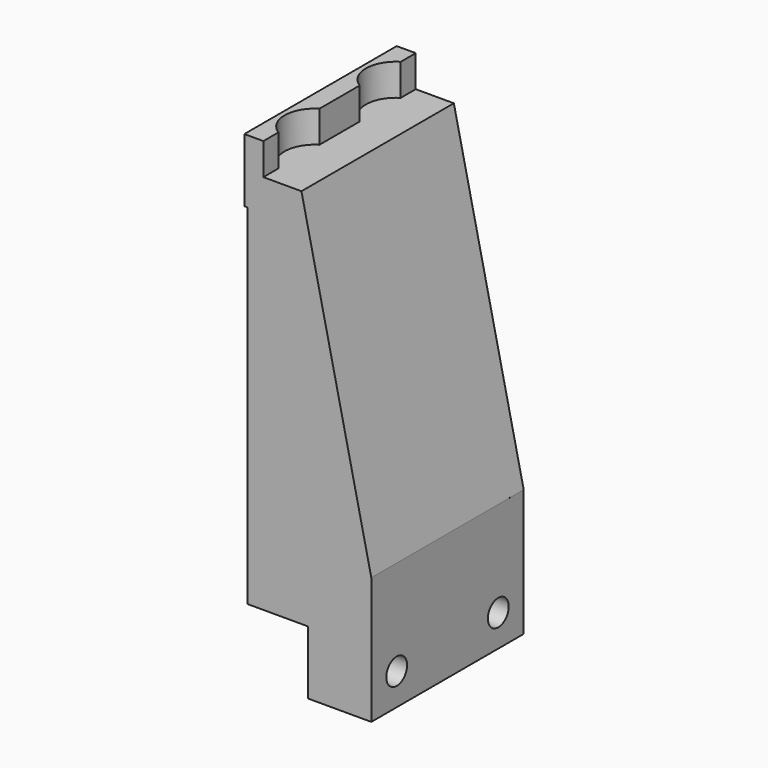
from build123d import *

# Parameters (mm, degrees)
F0_W      = 20
F0_H      = 70
F1_DEPTH  = 30
F2_W      = 30
F2_H      = 10
F3_DEPTH  = 10
F4_R      = 2.05
F5_DEPTH  = 10
F6_W      = 11
F6_H      = 30
F7_DEPTH  = 50
F9_DEPTH  = 5
F10_SIZE2 = 10.99999
F10_SIZE  = 49.99999
F11_W     = 30
F11_H     = 55
F12_DEPTH = 0.5


# Not quite as in the source:
# - a fillet or chamfer is up to 0.001 mm smaller than in the source, because OpenCascade refuses the exact size


with BuildPart() as f1:
    # F0 (on Front) → F1 (new body)
    with BuildSketch(Plane.XZ):
        with Locations((-10, 35)):
            Rectangle(F0_W, F0_H)
    extrude(amount=F1_DEPTH)

    # F2 (on face) → F3 (cut)
    with BuildSketch(Plane(origin=(-20, 0, 0), x_dir=(0, -1, 0), z_dir=(-1, 0, 0))):
        with Locations((15, 5)):
            Rectangle(F2_W, F2_H)
    extrude(amount=-F3_DEPTH, mode=Mode.SUBTRACT)

    # F4 (on face) → F5 (cut, through all)
    with BuildSketch(Plane(origin=(-10, 0, 0), x_dir=(0, -1, 0), z_dir=(-1, 0, 0))):
        with Locations((5, 5)):
            Circle(F4_R)
        with Locations((25, 5)):
            Circle(F4_R)
    extrude(amount=-F5_DEPTH, mode=Mode.SUBTRACT)

    # F6 (on face) → F7 (cut)
    with BuildSketch(Plane.XY.offset(70)):
        with Locations((-5.5, -15)):
            Rectangle(F6_W, F6_H)
    extrude(amount=-F7_DEPTH, mode=Mode.SUBTRACT)

    # F8 (on face) → F9 (join)
    with BuildSketch(Plane.XY.offset(70)):
        with BuildLine():
            ThreePointArc((-17, -11.0388736054), (-19.25, -7), (-17, -2.9611263946))
            Line((-17, -2.9611263946), (-17, 0))
            Line((-17, 0), (-20, 0))
            Line((-20, 0), (-20, -30))
            Line((-20, -30), (-17, -30))
            Line((-17, -30), (-17, -27.0388736054))
            ThreePointArc((-17, -27.0388736054), (-19.25, -23), (-17, -18.9611263946))
            Line((-17, -18.9611263946), (-17, -11.0388736054))
        make_face()
    extrude(amount=F9_DEPTH)

    # F10 (size 50 and 11 in the source; OpenCascade refuses exactly that, so slightly less here)
    f10_edges = [f1.edges().sort_by_distance(p)[0] for p in [
        (-11, -15, 20),
    ]]
    f10_side = f1.faces().sort_by_distance((-11, -15, 45))[0]
    chamfer(f10_edges, length=F10_SIZE, length2=F10_SIZE2, reference=f10_side)

    # F11 (on face) → F12 (cut)
    with BuildSketch(Plane(origin=(-20, 0, 0), x_dir=(0, -1, 0), z_dir=(-1, 0, 0))):
        with Locations((15, 37.5)):
            Rectangle(F11_W, F11_H)
    extrude(amount=-F12_DEPTH, mode=Mode.SUBTRACT)


solid = f1.part
